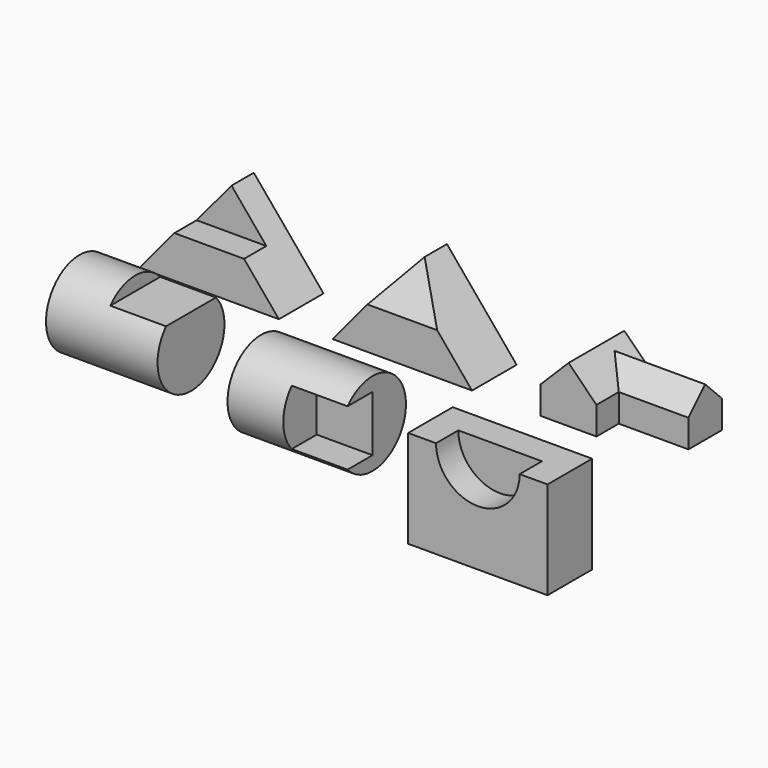
from build123d import *

# Parameters (mm, degrees)
F1_DEPTH  = 101.6
F3_DEPTH  = 50.8
F5_DEPTH  = 101.6
F9_DEPTH  = 76.2
F11_DEPTH = 127
F15_R     = 76.2
F16_DEPTH = 203.2
F18_DEPTH = 101.6
F20_R     = 76.2
F21_DEPTH = 203.2
F24_DEPTH = 101.6
F25_W     = 254
F25_H     = 177.8
F26_DEPTH = 101.6
F28_DEPTH = 50.8


with BuildPart() as f1:
    # F0 (on Front) → F1 (new body)
    with BuildSketch(Plane.XZ):
        Polygon((127, 152.4), (0, 0), (254, 0), align=None)
    extrude(amount=-F1_DEPTH)

    # F2 (on face) → F3 (cut)
    with BuildSketch(Plane.XZ):
        Polygon((127, 152.4), (63.5, 76.2), (190.5, 76.2), align=None)
    extrude(amount=-F3_DEPTH, mode=Mode.SUBTRACT)


with BuildPart() as f5:
    # F4 (on Front) → F5 (new body)
    with BuildSketch(Plane.XZ):
        Polygon((478.864695549, 152.4), (351.864695549, 0), (605.864695549, 0), align=None)
    extrude(amount=-F5_DEPTH)

    # F8 (on 3pt) → F9 (cut, symmetric)
    with BuildSketch(Plane.YZ.offset(478.864695549)):
        Polygon((0, 152.4), (0, 76.2), (50.8, 152.4), align=None)
    extrude(amount=F9_DEPTH, both=True, mode=Mode.SUBTRACT)


with BuildPart() as f11:
    # F10 (on Front) → F11 (new body)
    with BuildSketch(Plane.XZ):
        Polygon((730.9796256996, 50.8), (730.9796256996, 0), (832.5796256996, 0), (832.5796256996, 50.8), (781.7796256996, 101.6), align=None)
    extrude(amount=-F11_DEPTH)

    # F13 (on offset) → F14 (join, up to the next surface of F11)
    with BuildSketch(Plane.YZ.offset(959.5796256996)):
        Polygon((50.8, 50.8), (50.8, 0), (127, 0), (127, 50.8), (88.8999967435, 88.9), align=None)
    extrude(until=Until.NEXT, dir=(-1, 0, 0))


with BuildPart() as f16:
    # F15 (on Right) → F16 (new body)
    with BuildSketch(Plane.YZ):
        with Locations((-136.7214130477, 0)):
            Circle(F15_R)
    extrude(amount=F16_DEPTH)

    # F17 (on face) → F18 (cut)
    with BuildSketch(Plane.YZ.offset(203.2)):
        with BuildLine():
            ThreePointArc((-79.9252864192, 50.8), (-136.7214130477, 76.2), (-193.5175396762, 50.8))
            Line((-193.5175396762, 50.8), (-79.9252864192, 50.8))
        make_face()
    extrude(amount=-F18_DEPTH, mode=Mode.SUBTRACT)


with BuildPart() as f21:
    # F20 (on offset) → F21 (new body)
    with BuildSketch(Plane.YZ.offset(355.6)):
        with Locations((-167.850779579, 0)):
            Circle(F20_R)
    extrude(amount=F21_DEPTH)

    # F23 (on face) → F24 (cut)
    with BuildSketch(Plane.YZ.offset(558.8)):
        with BuildLine():
            Line((-167.850779579, 50.8), (-224.6469062075, 50.8))
            ThreePointArc((-224.6469062075, 50.8), (-244.050779579, 0), (-224.6469062075, -50.8))
            Line((-224.6469062075, -50.8), (-167.850779579, -50.8))
            Line((-167.850779579, -50.8), (-167.850779579, 50.8))
        make_face()
    extrude(amount=-F24_DEPTH, mode=Mode.SUBTRACT)


with BuildPart() as f26:
    # F25 (on offset) → F26 (new body)
    with BuildSketch(Plane.XZ.offset(226.06)):
        with Locations((878.5699307919, 23.7150967563)):
            Rectangle(F25_W, F25_H)
    extrude(amount=F26_DEPTH)

    # F27 (on face) → F28 (cut)
    with BuildSketch(Plane.XZ.offset(327.66)):
        with BuildLine():
            Line((802.3699307919, 112.6150967563), (954.7699307919, 112.6150967563))
            ThreePointArc((954.7699307919, 112.6150967563), (878.5699307919, 188.8150967563), (802.3699307919, 112.6150967563))
        make_face()
        with BuildLine():
            ThreePointArc((802.3699307919, 112.6150967563), (878.5699307919, 36.4150967563), (954.7699307919, 112.6150967563))
            Line((954.7699307919, 112.6150967563), (802.3699307919, 112.6150967563))
        make_face()
    extrude(amount=-F28_DEPTH, mode=Mode.SUBTRACT)


solid = Compound([f1.part, f5.part, f11.part, f16.part, f21.part, f26.part])
